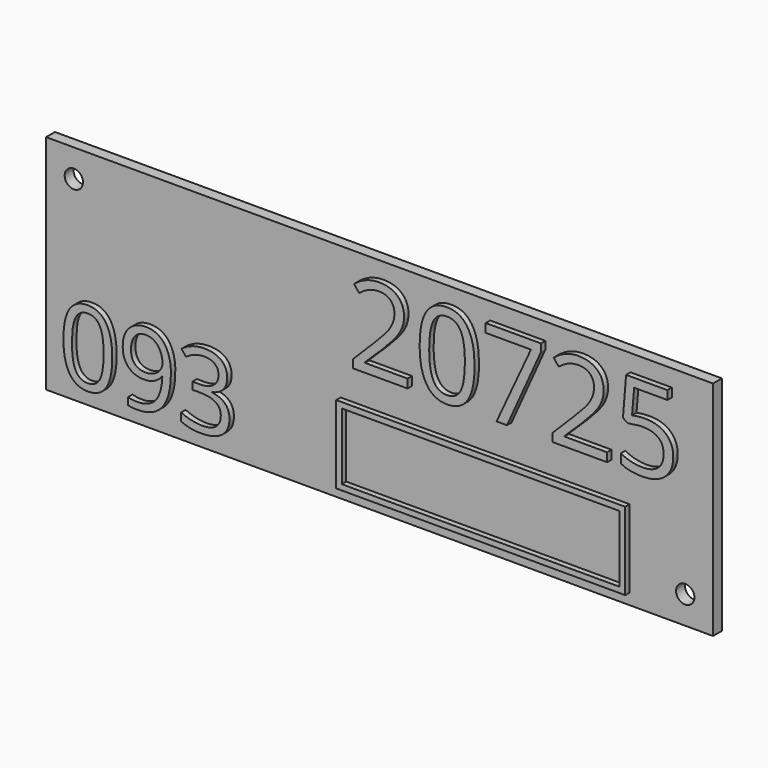
from build123d import *

# Parameters (mm, degrees)
F0_W         = 120
F0_H         = 40
F1_DEPTH     = 2
F3_D         = 3.3
F4_TEXT_SIZE = 20.9355577363
F5_DEPTH     = 1
F6_TEXT_SIZE = 18.5894526641
F7_DEPTH     = 1
F8_W         = 52
F8_H         = 14
F8_W_2       = 49.99999962
F8_H_2       = 11.99999962
F9_DEPTH     = 1


# Not quite as in the source:
# - Text() gives the source's letters only with a copy of the font that has no kerning and outlines rounded to 1/6400 em; it was checked with that copy


with BuildPart() as f1:
    # F0 (on Front) → F1 (new body)
    with BuildSketch(Plane.XZ):
        Rectangle(F0_W, F0_H)
    extrude(amount=F1_DEPTH)

    # F3 (through all)
    with Locations(Plane.XZ.offset(2)):
        with Locations((-55, 15), (55, -15)):
            Hole(F3_D / 2)

    # F4 (on face) → F5 (join)
    with BuildSketch(Plane.XZ.offset(2)):
        with Locations((-5, 2)):
            Text('20725', F4_TEXT_SIZE, font='Open Sans', text_align=(TextAlign.LEFT, TextAlign.BOTTOM))
    extrude(amount=F5_DEPTH)

    # F6 (on face) → F7 (join)
    with BuildSketch(Plane.XZ.offset(2)):
        with Locations((-57, -17)):
            Text('093', F6_TEXT_SIZE, font='Open Sans', text_align=(TextAlign.LEFT, TextAlign.BOTTOM))
    extrude(amount=F7_DEPTH)

    # F8 (on face) → F9 (join)
    with BuildSketch(Plane.XZ.offset(2)):
        with Locations((19, -11)):
            Rectangle(F8_W, F8_H)
        with Locations((19, -11)):
            Rectangle(F8_W_2, F8_H_2, mode=Mode.SUBTRACT)
    extrude(amount=F9_DEPTH)


solid = f1.part
